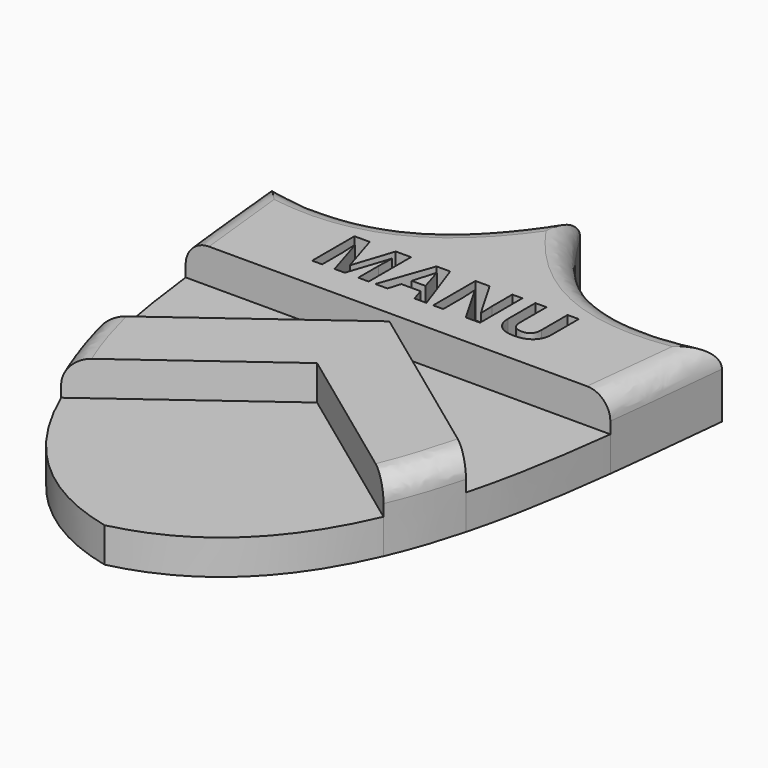
from build123d import *

# Parameters (mm, degrees)
F1_DEPTH     = 15.24
F2_DEPTH     = 7.62
F3_TEXT_SIZE = 16.254106433
F4_DEPTH     = 7.62
F5_R         = 5.08


# Not quite as in the source:
# - Text() gives the source's letters only with a copy of the font that has no kerning and outlines rounded to 1/6400 em; it was checked with that copy


with BuildPart() as f1:
    # F0 (on Top) → F1 (new body)
    with BuildSketch(Plane.XY):
        with BuildLine():
            add(Edge.make_bspline(
                [(-49.4390167296, 33.3175957203), (-23.4059114009, 26.3913571835), (-10.5087757111, 38.5719835758), (0, 56.2458336353)],
                knots=[0, 0, 0, 0, 54.4969766967, 54.4969766967, 54.4969766967, 54.4969766967], degree=3))
            add(Edge.make_bspline(
                [(-49.4390167296, 33.3175957203), (-48.5311618187, 24.8947121068), (-47.7085143411, 15.6836564118), (-46.5729604787, 6.2984688145)],
                knots=[0, 0, 0, 0, 24.9825344568, 24.9825344568, 24.9825344568, 24.9825344568], degree=3))
            Line((-46.5729604787, 6.2984688145), (0, 6.2984688145))
            Line((0, 6.2984688145), (46.5729604787, 6.2984688145))
            add(Edge.make_bspline(
                [(49.4390167296, 33.3175957203), (48.5311618187, 24.8947121068), (47.7085143411, 15.6836564118), (46.5729604787, 6.2984688145)],
                knots=[0, 0, 0, 0, 24.9825344568, 24.9825344568, 24.9825344568, 24.9825344568], degree=3))
            add(Edge.make_bspline(
                [(49.4390167296, 33.3175957203), (23.4059114009, 26.3913571835), (10.5087757111, 38.5719835758), (0, 56.2458336353)],
                knots=[0, 0, 0, 0, 54.4969766967, 54.4969766967, 54.4969766967, 54.4969766967], degree=3))
        make_face()
    extrude(amount=F1_DEPTH)



with BuildPart() as f1b:
    # F0 (on Top) → F1, piece 2 (new body)
    with BuildSketch(Plane.XY):
        with BuildLine():
            Line((0, 3.9407913573), (-40.7607806818, -26.0162340737))
            add(Edge.make_bspline(
                [(-40.7607806818, -26.0162340737), (-39.2840975767, -31.5516400573), (-37.5126704202, -36.8827349338), (-35.3528329599, -41.8650503634)],
                knots=[53.8784554206, 53.8784554206, 53.8784554206, 53.8784554206, 69.3012044919, 69.3012044919, 69.3012044919, 69.3012044919], degree=3))
            Line((-35.3528329599, -41.8650503634), (0, -15.8825814724))
            Line((0, -15.8825814724), (35.3528329599, -41.8650503634))
            add(Edge.make_bspline(
                [(40.7607806818, -26.0162340737), (39.2840975767, -31.5516400573), (37.5126704202, -36.8827349338), (35.3528329599, -41.8650503634)],
                knots=[53.8784554206, 53.8784554206, 53.8784554206, 53.8784554206, 69.3012044919, 69.3012044919, 69.3012044919, 69.3012044919], degree=3))
            Line((40.7607806818, -26.0162340737), (0, 3.9407913573))
        make_face()
    extrude(amount=F1_DEPTH)


with BuildPart() as f1_1:
    add(f1.part)

    add(f1b.part)  # F2 merges F1b
    # F0 (on Top) → F2 (join)
    with BuildSketch(Plane.XY):
        with BuildLine():
            add(Edge.make_bspline(
                [(-49.4390167296, 33.3175957203), (-23.4059114009, 26.3913571835), (-10.5087757111, 38.5719835758), (0, 56.2458336353)],
                knots=[0, 0, 0, 0, 54.4969766967, 54.4969766967, 54.4969766967, 54.4969766967], degree=3))
            add(Edge.make_bspline(
                [(-49.4390167296, 33.3175957203), (-48.5311618187, 24.8947121068), (-47.7085143411, 15.6836564118), (-46.5729604787, 6.2984688145)],
                knots=[0, 0, 0, 0, 24.9825344568, 24.9825344568, 24.9825344568, 24.9825344568], degree=3))
            Line((-46.5729604787, 6.2984688145), (0, 6.2984688145))
            Line((0, 6.2984688145), (46.5729604787, 6.2984688145))
            add(Edge.make_bspline(
                [(49.4390167296, 33.3175957203), (48.5311618187, 24.8947121068), (47.7085143411, 15.6836564118), (46.5729604787, 6.2984688145)],
                knots=[0, 0, 0, 0, 24.9825344568, 24.9825344568, 24.9825344568, 24.9825344568], degree=3))
            add(Edge.make_bspline(
                [(49.4390167296, 33.3175957203), (23.4059114009, 26.3913571835), (10.5087757111, 38.5719835758), (0, 56.2458336353)],
                knots=[0, 0, 0, 0, 54.4969766967, 54.4969766967, 54.4969766967, 54.4969766967], degree=3))
        make_face()
        with BuildLine():
            Line((0, 6.2984688145), (-46.5729604787, 6.2984688145))
            add(Edge.make_bspline(
                [(-46.5729604787, 6.2984688145), (-45.2595278997, -4.5568605161), (-43.5274805806, -15.6451482793), (-40.7607806818, -26.0162340737)],
                knots=[24.9825344568, 24.9825344568, 24.9825344568, 24.9825344568, 53.8784554206, 53.8784554206, 53.8784554206, 53.8784554206], degree=3))
            Line((-40.7607806818, -26.0162340737), (0, 3.9407913573))
            Line((0, 3.9407913573), (40.7607806818, -26.0162340737))
            add(Edge.make_bspline(
                [(46.5729604787, 6.2984688145), (45.2595278997, -4.5568605161), (43.5274805806, -15.6451482793), (40.7607806818, -26.0162340737)],
                knots=[24.9825344568, 24.9825344568, 24.9825344568, 24.9825344568, 53.8784554206, 53.8784554206, 53.8784554206, 53.8784554206], degree=3))
            Line((46.5729604787, 6.2984688145), (0, 6.2984688145))
        make_face()
        with BuildLine():
            Line((0, 3.9407913573), (-40.7607806818, -26.0162340737))
            add(Edge.make_bspline(
                [(-40.7607806818, -26.0162340737), (-39.2840975767, -31.5516400573), (-37.5126704202, -36.8827349338), (-35.3528329599, -41.8650503634)],
                knots=[53.8784554206, 53.8784554206, 53.8784554206, 53.8784554206, 69.3012044919, 69.3012044919, 69.3012044919, 69.3012044919], degree=3))
            Line((-35.3528329599, -41.8650503634), (0, -15.8825814724))
            Line((0, -15.8825814724), (35.3528329599, -41.8650503634))
            add(Edge.make_bspline(
                [(40.7607806818, -26.0162340737), (39.2840975767, -31.5516400573), (37.5126704202, -36.8827349338), (35.3528329599, -41.8650503634)],
                knots=[53.8784554206, 53.8784554206, 53.8784554206, 53.8784554206, 69.3012044919, 69.3012044919, 69.3012044919, 69.3012044919], degree=3))
            Line((40.7607806818, -26.0162340737), (0, 3.9407913573))
        make_face()
        with BuildLine():
            Line((0, -15.8825814724), (-35.3528329599, -41.8650503634))
            add(Edge.make_bspline(
                [(-35.3528329599, -41.8650503634), (-28.4906658817, -57.6947049292), (-17.70773049, -70.0036408354), (0, -74.158526957)],
                knots=[69.3012044919, 69.3012044919, 69.3012044919, 69.3012044919, 118.3018737, 118.3018737, 118.3018737, 118.3018737], degree=3))
            add(Edge.make_bspline(
                [(35.3528329599, -41.8650503634), (28.4906658817, -57.6947049292), (17.70773049, -70.0036408354), (0, -74.158526957)],
                knots=[69.3012044919, 69.3012044919, 69.3012044919, 69.3012044919, 118.3018737, 118.3018737, 118.3018737, 118.3018737], degree=3))
            Line((35.3528329599, -41.8650503634), (0, -15.8825814724))
        make_face()
    extrude(amount=F2_DEPTH)

    # F3 (on face) → F4 (cut)
    with BuildSketch(Plane.XY.offset(15.24)):
        with Locations((-25.8567277492, 13.2553875446)):
            Text('MANU', F3_TEXT_SIZE, font='Open Sans', font_style=FontStyle.BOLD, text_align=(TextAlign.LEFT, TextAlign.BOTTOM))
    extrude(amount=-F4_DEPTH, mode=Mode.SUBTRACT)

    # F5
    f5_edges = [f1_1.edges().sort_by_distance(p)[0] for p in [
        (-38.349244, -34.040923, 15.24),
        (38.349244, -34.040923, 15.24),
        (48.05407, 19.802842, 15.24),
        (-48.05407, 19.802842, 15.24),
        (-20.263578, 34.829432, 15.24),
        (20.263578, 34.829432, 15.24),
    ]]
    fillet(f5_edges, radius=F5_R)


solid = f1_1.part
